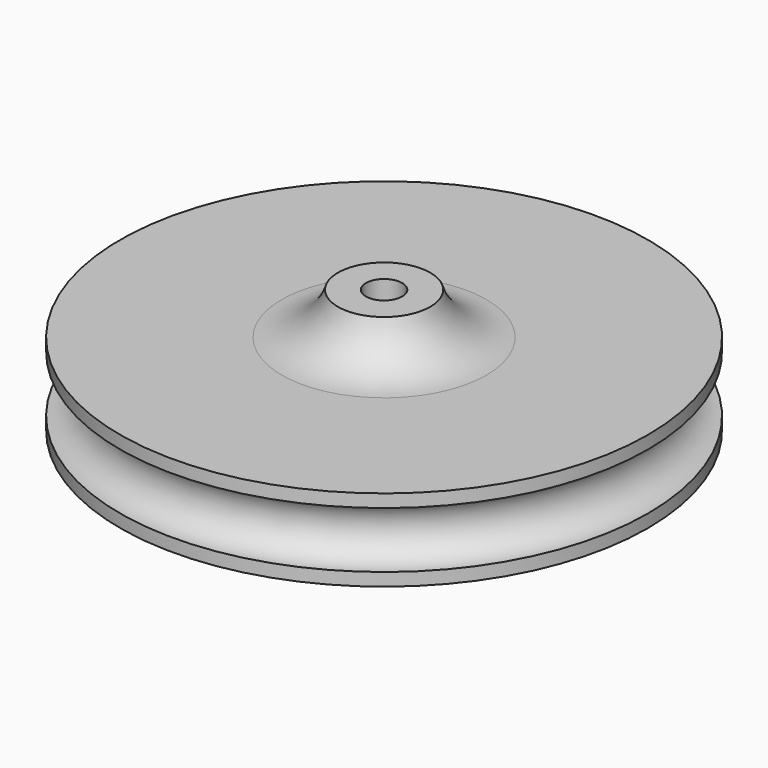
from build123d import *


# Not quite as in the source:
# - a fillet or chamfer that OpenCascade refuses, or shapes differently, is made with other operations: its cross-section is extruded or revolved along the edge and cut away or added
# - ends of sketch curves that miss each other by under 0.0002 mm in the source are joined


with BuildPart() as f1:
    # F0 (on Front) → F1 (revolve)
    with BuildSketch(Plane.XZ):
        with BuildLine():
            Line((1.55, 10.5700949207), (1.55, 4.9207e-06))
            Line((1.55, 4.9207e-06), (22.5, 0))
            Line((22.5, 0), (22.5, 1.1))
            ThreePointArc((22.5, 1.1), (20.1, 3.5), (22.5, 5.9))
            Line((22.5, 5.9), (22.5, 7))
            Line((22.5, 7), (3.9362940006, 7))
            Line((3.9362940006, 7), (3.9362940006, 10.5700949207))
            Line((3.9362940006, 10.5700949207), (1.55, 10.5700949207))
        make_face()
    revolve(axis=Axis((0, 0, 5.2850474603), (0, 0, -1)))

    # F2: fillet of radius 5 on 1 edges, made by hand

    # F2_s1 → F2_t2 (revolve)
    with BuildSketch(Plane.XZ):
        with BuildLine():
            ThreePointArc((8.7274704182, 7), (5.739956853, 7.9906655542), (3.9362940006, 10.5700949207))
            Line((3.9362940006, 10.5700949207), (3.9362940006, 7))
            Line((3.9362940006, 7), (8.7274704182, 7))
        make_face()
    revolve(axis=Axis((0, 0, 7), (0, 0, -1)))


solid = f1.part
